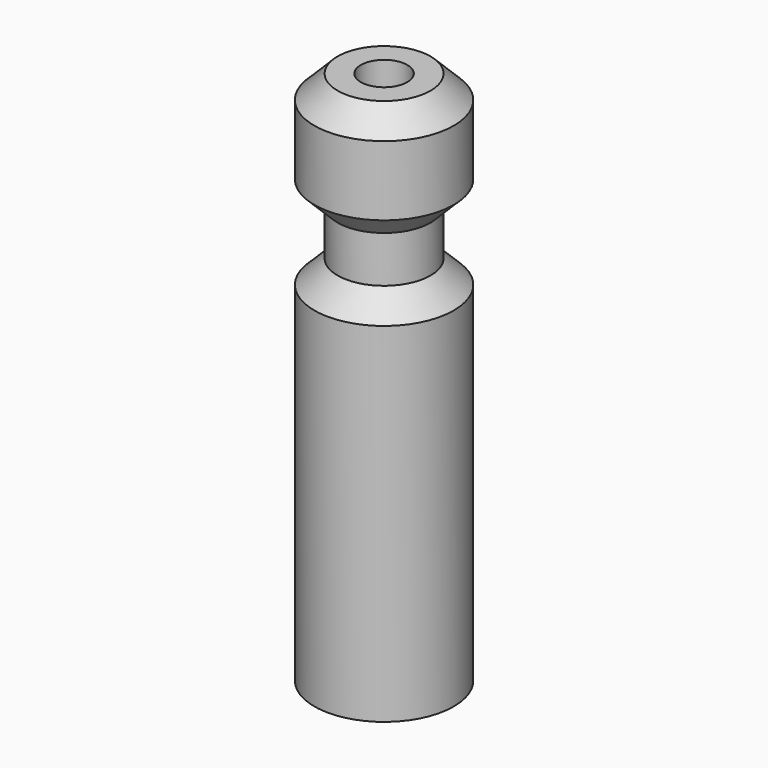
from build123d import *

# Parameters (mm, degrees)
F0_R     = 3
F1_DEPTH = 16
F2_R     = 2
F3_DEPTH = 2
F4_R     = 3
F5_DEPTH = 5
F6_SIZE  = 0.99999
F7_R     = 1
F8_DEPTH = 25


# Not quite as in the source:
# - a fillet or chamfer is up to 0.001 mm smaller than in the source, because OpenCascade refuses the exact size


with BuildPart() as f1:
    # F0 (on Top) → F1 (new body)
    with BuildSketch(Plane.XY):
        Circle(F0_R)
    extrude(amount=F1_DEPTH)

    # F2 (on face) → F3 (join)
    with BuildSketch(Plane.XY.offset(16)):
        Circle(F2_R)
    extrude(amount=F3_DEPTH)

    # F4 (on face) → F5 (join)
    with BuildSketch(Plane.XY.offset(18)):
        Circle(F4_R)
    extrude(amount=F5_DEPTH)

    # F6 (size 1 in the source; OpenCascade refuses exactly that, so slightly less here)
    f6_edges = [f1.edges().sort_by_distance(p)[0] for p in [
        (-3, 0, 23),
        (-3, 0, 18),
        (-3, 0, 16),
    ]]
    chamfer(f6_edges, length=F6_SIZE)

    # F7 (on face) → F8 (cut)
    with BuildSketch(Plane(origin=(0, 0, 0), x_dir=(1, 0, 0), z_dir=(0, 0, -1))):
        Circle(F7_R)
    extrude(amount=-F8_DEPTH, mode=Mode.SUBTRACT)


solid = f1.part
